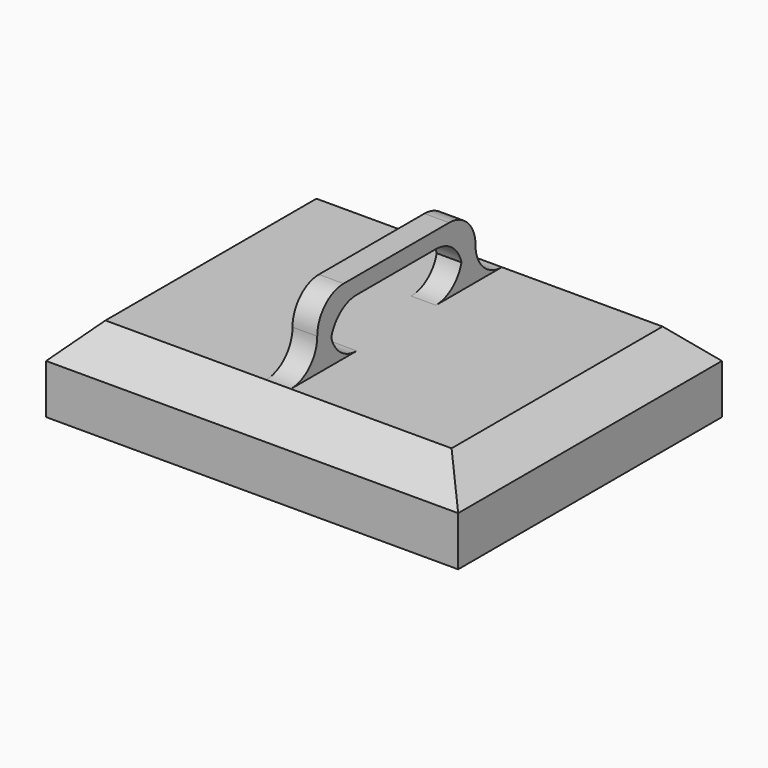
from build123d import *

# Parameters (mm, degrees)
F0_W        = 25
F0_H        = 20
F1_DEPTH    = 5
F3_DEPTH    = 0.75
F4_T1_DEPTH = 1.5
F4_T3_DEPTH = 11.5
F5_SIZE     = 1.99999


# Not quite as in the source:
# - a fillet or chamfer that OpenCascade refuses, or shapes differently, is made with other operations: its cross-section is extruded or revolved along the edge and cut away or added
# - a fillet or chamfer is up to 0.001 mm smaller than in the source, because OpenCascade refuses the exact size


with BuildPart() as f1:
    # F0 (on Top) → F1 (new body)
    with BuildSketch(Plane.XY):
        Rectangle(F0_W, F0_H)
    extrude(amount=-F1_DEPTH)

    # F2 (on Right) → F3 (join, symmetric)
    with BuildSketch(Plane.YZ):
        Polygon((-6, 4), (-6, 0), (-5, 0), (-5, 3), (5, 3), (5, 0), (6, 0), (6, 4), align=None)
    extrude(amount=F3_DEPTH, both=True)

    # F4: fillet of radius 2 on 8 edges, made by hand

    # F4_s2 → F4_t1 (join)
    with BuildSketch(Plane.YZ.offset(-0.75)):
        with BuildLine():
            ThreePointArc((-3, 0), (-4.4142135624, 0.5857864376), (-5, 2))
            Line((-5, 2), (-5, 0))
            Line((-5, 0), (-3, 0))
        make_face()
        with BuildLine():
            ThreePointArc((3, 0), (4.4142135624, 0.5857864376), (5, 2))
            Line((5, 2), (5, 0))
            Line((5, 0), (3, 0))
        make_face()
        with BuildLine():
            ThreePointArc((-8, 0), (-6.5857864376, 0.5857864376), (-6, 2))
            Line((-6, 2), (-6, 0))
            Line((-6, 0), (-8, 0))
        make_face()
        with BuildLine():
            ThreePointArc((8, 0), (6.5857864376, 0.5857864376), (6, 2))
            Line((6, 2), (6, 0))
            Line((6, 0), (8, 0))
        make_face()
        with BuildLine():
            ThreePointArc((-5, 1), (-4.4142135624, 2.4142135624), (-3, 3))
            Line((-3, 3), (-5, 3))
            Line((-5, 3), (-5, 1))
        make_face()
        with BuildLine():
            ThreePointArc((5, 1), (4.4142135624, 2.4142135624), (3, 3))
            Line((3, 3), (5, 3))
            Line((5, 3), (5, 1))
        make_face()
    extrude(amount=F4_T1_DEPTH)

    # F4_s4 → F4_t3 (cut)
    with BuildSketch(Plane.YZ.offset(-5.75)):
        with BuildLine():
            ThreePointArc((-4, 4), (-5.4142135624, 3.4142135624), (-6, 2))
            Line((-6, 2), (-6, 4))
            Line((-6, 4), (-4, 4))
        make_face()
        with BuildLine():
            ThreePointArc((6, 2), (5.4142135624, 3.4142135624), (4, 4))
            Line((4, 4), (6, 4))
            Line((6, 4), (6, 2))
        make_face()
    extrude(amount=F4_T3_DEPTH, mode=Mode.SUBTRACT)

    # F5 (size 2 in the source; OpenCascade refuses exactly that, so slightly less here)
    f5_edges = [f1.edges().sort_by_distance(p)[0] for p in [
        (12.5, 0, 0),
        (0, -10, 0),
        (0, 10, 0),
        (-12.5, 0, 0),
    ]]
    chamfer(f5_edges, length=F5_SIZE)


solid = f1.part
